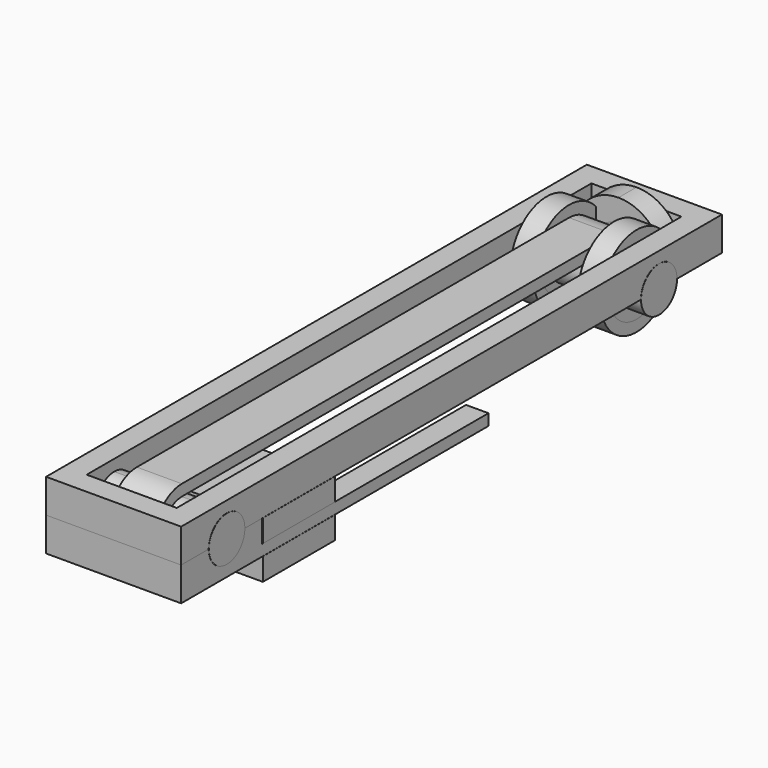
from build123d import *

# Parameters (mm, degrees)
F2_DEPTH  = 6.35
F3_R      = 12.7
F3_R_2    = 9.525
F4_DEPTH  = 12.7
F5_DEPTH  = 6.35
F3_R_3    = 6.35
F6_DEPTH  = 19.05
F7_DEPTH  = 12.7
F8_DEPTH  = 6.35
F10_DEPTH = 6.35
F11_DEPTH = 19.05
F9_W      = 25.4
F9_H      = 6.35
F12_DEPTH = 19.05
F13_DEPTH = 6.35
F15_W     = 6.3629296671
F15_H     = 79.796386
F15_W_2   = 6.3370703329
F16_DEPTH = 9.525
F17_DEPTH = 6.35
F18_DEPTH = 9.525


# Not quite as in the source:
# - a feature names something its author has since deleted; it is built from what else it names


with BuildPart() as f2:
    # F1 (on offset) → F2 (new body)
    with BuildSketch(Plane.XZ.offset(28.575)):
        with BuildLine():
            ThreePointArc((12.7, -25.4), (8.9802561211, -16.4197438789), (0, -12.7))
            ThreePointArc((0, -12.7), (-8.9802561211, -34.3802561211), (12.7, -25.4))
        make_face()
        with BuildLine():
            ThreePointArc((6.35, -25.4), (-4.4901280605, -29.8901280605), (0, -19.05))
            ThreePointArc((0, -19.05), (4.4901280605, -20.9098719395), (6.35, -25.4))
        make_face(mode=Mode.SUBTRACT)
    extrude(amount=F2_DEPTH)


with BuildPart() as f4:
    # F3 (on Right) → F4 (new body, symmetric)
    with BuildSketch(Plane.YZ):
        with Locations((-44.45, -25.4)):
            Circle(F3_R)
        with Locations((-44.45, -25.4)):
            Circle(F3_R_2, mode=Mode.SUBTRACT)
    extrude(amount=F4_DEPTH, both=True)

    # F3 (on Right) → F5 (cut, symmetric)
    with BuildSketch(Plane.YZ):
        with Locations((-44.45, -25.4)):
            Circle(F3_R)
        with Locations((-44.45, -25.4)):
            Circle(F3_R_2, mode=Mode.SUBTRACT)
    extrude(amount=F5_DEPTH, both=True, mode=Mode.SUBTRACT)


with BuildPart() as f6:
    # F3 (on Right) → F6 (new body, symmetric)
    with BuildSketch(Plane.YZ):
        with Locations((-44.45, -25.4)):
            Circle(F3_R_3)
    extrude(amount=F6_DEPTH, both=True)


with BuildPart() as f7:
    # F3 (on Right) → F7 (new body, symmetric)
    with BuildSketch(Plane.YZ):
        with Locations((-44.45, -25.4)):
            Circle(F3_R_2)
        with Locations((-44.45, -25.4)):
            Circle(F3_R_3, mode=Mode.SUBTRACT)
    extrude(amount=F7_DEPTH, both=True)

    # F3 (on Right) → F8 (cut, symmetric)
    with BuildSketch(Plane.YZ):
        with Locations((-44.45, -25.4)):
            Circle(F3_R_2)
        with Locations((-44.45, -25.4)):
            Circle(F3_R_3, mode=Mode.SUBTRACT)
    extrude(amount=F8_DEPTH, both=True, mode=Mode.SUBTRACT)


with BuildPart() as f10:
    # F9 (on Right) → F10 (new body, symmetric)
    with BuildSketch(Plane.YZ):
        with BuildLine():
            Line((-158.75, -34.925), (-44.45, -34.925))
            ThreePointArc((-44.45, -34.925), (-34.925, -25.4), (-44.45, -15.875))
            Line((-44.45, -15.875), (-196.85, -15.875))
            ThreePointArc((-196.85, -15.875), (-206.375, -25.4), (-196.85, -34.925))
            Line((-196.85, -34.925), (-184.15, -34.925))
            Line((-184.15, -34.925), (-158.75, -34.925))
        make_face()
        with BuildLine():
            ThreePointArc((-44.45, -19.05), (-39.9598719395, -20.9098719395), (-38.1, -25.4))
            ThreePointArc((-38.1, -25.4), (-39.9598719395, -29.8901280605), (-44.45, -31.75))
            Line((-44.45, -31.75), (-158.75, -31.75))
            Line((-158.75, -31.75), (-184.15, -31.75))
            Line((-184.15, -31.75), (-196.85, -31.75))
            ThreePointArc((-196.85, -31.75), (-203.2, -25.4), (-196.85, -19.05))
            Line((-196.85, -19.05), (-44.45, -19.05))
        make_face(mode=Mode.SUBTRACT)
    extrude(amount=F10_DEPTH, both=True)


with BuildPart() as f11:
    # F9 (on Right) → F11 (new body, symmetric)
    with BuildSketch(Plane.YZ):
        with BuildLine():
            ThreePointArc((-190.5, -25.4), (-192.3598719395, -20.9098719395), (-196.85, -19.05))
            ThreePointArc((-196.85, -19.05), (-203.2, -25.4), (-196.85, -31.75))
            ThreePointArc((-196.85, -31.75), (-192.3598719395, -29.8901280605), (-190.5, -25.4))
        make_face()
    extrude(amount=F11_DEPTH, both=True)


with BuildPart() as f12:
    # F9 (on Right) → F12 (new body, symmetric)
    with BuildSketch(Plane.YZ):
        with Locations((-171.45, -28.575)):
            Rectangle(F9_W, F9_H)
    extrude(amount=F12_DEPTH, both=True)


with BuildPart() as f12b:
    # F9 (on Right) → F12, piece 2 (new body, symmetric)
    with BuildSketch(Plane.YZ):
        with Locations((-171.45, -38.1)):
            Rectangle(F9_W, F9_H)
    extrude(amount=F12_DEPTH, both=True)


with BuildPart() as f13:
    # F1 (on offset) → F13 (new body, symmetric)
    with BuildSketch(Plane.XZ.offset(28.575)):
        with BuildLine():
            ThreePointArc((6.35, -25.4), (4.4901280605, -20.9098719395), (0, -19.05))
            ThreePointArc((0, -19.05), (-4.4901280605, -29.8901280605), (6.35, -25.4))
        make_face()
    extrude(amount=F13_DEPTH, both=True)


with BuildPart() as f16:
    # F15 (on offset) → F16 (new body)
    with BuildSketch(Plane.XY.offset(-25.4)):
        Polygon((-19.0887890014, -184.3439450068), (-19.0887890014, -212.9189450068), (19.0112109986, -212.9189450068), (19.0112109986, -184.3439450068), (12.6741406658, -184.3439450068), (12.6741406658, -206.5560153396), (-12.7258593342, -206.5560153396), (-12.7258593342, -184.3439450068), align=None)
        with Locations((-15.9073241678, -144.4457520068)):
            Rectangle(F15_W, F15_H)
        with Locations((15.8426758322, -144.4457520068)):
            Rectangle(F15_W_2, F15_H)
    extrude(amount=-F16_DEPTH)

    # F15 (on offset) → F17 (cut)
    with BuildSketch(Plane.XY.offset(-25.4)):
        with Locations((-15.9073241678, -144.4457520068)):
            Rectangle(F15_W, F15_H)
        with Locations((15.8426758322, -144.4457520068)):
            Rectangle(F15_W_2, F15_H)
    extrude(amount=-F17_DEPTH, mode=Mode.SUBTRACT)

    # F19: cut F11, F6, F13
    add(f11.part, mode=Mode.SUBTRACT)
    add(f6.part, mode=Mode.SUBTRACT)
    add(f13.part, mode=Mode.SUBTRACT)


with BuildPart() as f18:
    # F15 (on offset) → F18 (new body)
    with BuildSketch(Plane.XY.offset(-25.4)):
        Polygon((-19.0887890014, -184.3439450068), (-19.0887890014, -212.9189450068), (19.0112109986, -212.9189450068), (19.0112109986, -184.3439450068), (12.6741406658, -184.3439450068), (12.6741406658, -206.5560153396), (-12.7258593342, -206.5560153396), (-12.7258593342, -184.3439450068), align=None)
        Polygon((-19.0887890014, -22.225), (-19.0887890014, -104.5475590068), (-12.7258593342, -104.5475590068), (-12.7258593342, -28.575), (-12.7, -28.575), (12.6741406658, -28.575), (12.6741406658, -104.5475590068), (19.0112109986, -104.5475590068), (19.0112109986, -22.225), align=None)
        with Locations((-15.9073241678, -144.4457520068)):
            Rectangle(F15_W, F15_H)
        with Locations((15.8426758322, -144.4457520068)):
            Rectangle(F15_W_2, F15_H)
    extrude(amount=F18_DEPTH)

    # F19: cut F11, F6, F13
    add(f11.part, mode=Mode.SUBTRACT)
    add(f6.part, mode=Mode.SUBTRACT)
    add(f13.part, mode=Mode.SUBTRACT)


solid = Compound([f2.part, f4.part, f6.part, f7.part, f10.part, f11.part, f12.part, f12b.part, f13.part, f16.part, f18.part])
